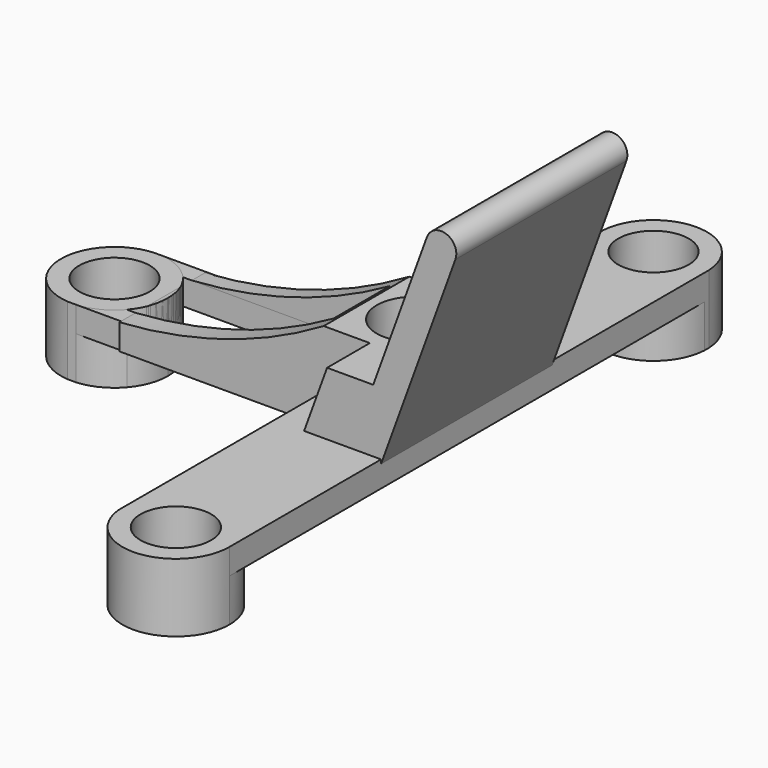
from build123d import *

# Parameters (mm, degrees)
F0_R      = 2.286
F0_R_2    = 2.0955
F2_DEPTH  = 1.524
F3_DEPTH  = 6.35
F4_DEPTH  = 3.175
F5_DEPTH  = 1.524
F6_DEPTH  = 12.7
F0_R_3    = 0.8255
F7_DEPTH  = 2.54
F8_DEPTH  = 1.524
F9_DEPTH  = 2.54
F10_DEPTH = 1.524
F11_DEPTH = 2.54
F12_DEPTH = 1.524
F13_DEPTH = 25.4


with BuildPart() as f2:
    # F0 (on Top) → F2 (new body)
    with BuildSketch(Plane.XY):
        with BuildLine():
            Line((4.9948175588, 3.2833689949), (4.9948175588, 2.2014643259))
            Line((4.9948175588, 2.2014643259), (4.9948175588, -1.9667148894))
            Line((4.9948175588, -1.9667148894), (4.9948175588, -3.0515958757))
            Line((4.9948175588, -3.0515958757), (4.9948175588, -17.3166585326))
            ThreePointArc((4.9948175588, -17.3166585326), (8.3062650536, -14.4464316119), (11.3304992405, -17.6178500122))
            Line((11.3304992405, -17.6178500122), (11.3304992405, 17.6788508391))
            ThreePointArc((11.3304992405, 17.6788508391), (8.2060050581, 14.6658888438), (4.9948175588, 17.5862790105))
            Line((4.9948175588, 17.5862790105), (4.9948175588, 3.2833689949))
        make_face()
        with Locations((8.2809459418, 0)):
            Circle(F0_R, mode=Mode.SUBTRACT)
        with BuildLine():
            Line((4.9948175588, 18.0948209651), (4.9948175588, 17.5862790105))
            ThreePointArc((4.9948175588, 17.5862790105), (8.2060050581, 14.6658888438), (11.3304992405, 17.6788508391))
            Line((11.3304992405, 17.6788508391), (11.3304992405, 18.0022491365))
            ThreePointArc((11.3304992405, 18.0022491365), (8.2060050581, 21.0152111318), (4.9948175588, 18.0948209651))
        make_face()
        with Locations((8.1596194911, 17.8405499878)):
            Circle(F0_R_2, mode=Mode.SUBTRACT)
        with BuildLine():
            ThreePointArc((11.3304992405, -17.6178500122), (8.3062650536, -14.4464316119), (4.9948175588, -17.3166585326))
            Line((4.9948175588, -17.3166585326), (4.9948175588, -17.9190414918))
            ThreePointArc((4.9948175588, -17.9190414918), (8.3062650536, -20.7892684125), (11.3304992405, -17.6178500122))
        make_face()
        with Locations((8.1554992405, -17.6178500122)):
            Circle(F0_R_2, mode=Mode.SUBTRACT)
    extrude(amount=F2_DEPTH)

    # F1 (on Front) → F3 (join, symmetric)
    with BuildSketch(Plane.XZ):
        with BuildLine():
            Line((10.8624471896, 5.2727888553), (8.1229047444, 5.2727888553))
            Line((8.1229047444, 5.2727888553), (6.2037665495, 0))
            Line((6.2037665495, 0), (10.8624471896, 0))
            Line((10.8624471896, 0), (15.7450092285, 13.4147289508))
            ThreePointArc((15.7450092285, 13.4147289508), (15.2060879556, 14.5704493502), (14.0503675562, 14.0315280773))
            Line((14.0503675562, 14.0315280773), (10.8624471896, 5.2727888553))
        make_face()
    extrude(amount=F3_DEPTH, both=True)

    # F1 (on Front) → F4 (join, symmetric)
    with BuildSketch(Plane.XZ):
        with BuildLine():
            Line((8.1229047444, 5.2727888553), (5.3833622992, 5.2727888553))
            ThreePointArc((5.3833622992, 5.2727888553), (-0.4659601575, 2.6817210776), (-6.7578507587, 1.524))
            Line((-6.7578507587, 1.524), (-6.7578507587, 0))
            Line((-6.7578507587, 0), (5.0566992405, 0))
            Line((5.0566992405, 0), (6.2037665495, 0))
            Line((6.2037665495, 0), (8.1229047444, 5.2727888553))
        make_face()
    extrude(amount=F4_DEPTH, both=True)

    # F0 (on Top) → F6 (cut, symmetric)
    with BuildSketch(Plane.XY):
        with BuildLine():
            ThreePointArc((-7.2838490429, 2.2014643259), (-6.7026349357, 1.2283188177), (-6.5003007595, 0.1130238343))
            ThreePointArc((-6.5003007595, 0.1130238343), (-6.7006139401, -0.9968695509), (-7.2762776581, -1.9667148894))
            Line((-7.2762776581, -1.9667148894), (4.9948175588, -1.9667148894))
            Line((4.9948175588, -1.9667148894), (4.9948175588, 2.2014643259))
            Line((4.9948175588, 2.2014643259), (-7.2838490429, 2.2014643259))
        make_face()
    extrude(amount=F6_DEPTH, both=True, mode=Mode.SUBTRACT)

    # F0 (on Top) → F7 (join)
    with BuildSketch(Plane.XY):
        with BuildLine():
            ThreePointArc((11.3304992405, -17.6178500122), (8.3062650536, -14.4464316119), (4.9948175588, -17.3166585326))
            Line((4.9948175588, -17.3166585326), (4.9948175588, -17.9190414918))
            ThreePointArc((4.9948175588, -17.9190414918), (8.3062650536, -20.7892684125), (11.3304992405, -17.6178500122))
        make_face()
        with Locations((8.1554992405, -17.6178500122)):
            Circle(F0_R_2, mode=Mode.SUBTRACT)
        with Locations((8.1554992405, -17.6178500122)):
            Circle(F0_R_2)
        with Locations((8.1554992405, -17.6178500122)):
            Circle(F0_R_3, mode=Mode.SUBTRACT)
    extrude(amount=-F7_DEPTH)

    # F0 (on Top) → F8 (cut)
    with BuildSketch(Plane.XY):
        with Locations((8.1554992405, -17.6178500122)):
            Circle(F0_R_2)
        with Locations((8.1554992405, -17.6178500122)):
            Circle(F0_R_3, mode=Mode.SUBTRACT)
    extrude(amount=-F8_DEPTH, mode=Mode.SUBTRACT)

    # F0 (on Top) → F11 (join)
    with BuildSketch(Plane.XY):
        with BuildLine():
            Line((4.9948175588, 18.0948209651), (4.9948175588, 17.5862790105))
            ThreePointArc((4.9948175588, 17.5862790105), (8.2060050581, 14.6658888438), (11.3304992405, 17.6788508391))
            Line((11.3304992405, 17.6788508391), (11.3304992405, 18.0022491365))
            ThreePointArc((11.3304992405, 18.0022491365), (8.2060050581, 21.0152111318), (4.9948175588, 18.0948209651))
        make_face()
        with Locations((8.1596194911, 17.8405499878)):
            Circle(F0_R_2, mode=Mode.SUBTRACT)
        with Locations((8.1596194911, 17.8405499878)):
            Circle(F0_R_2)
        with Locations((8.1596194911, 17.8405499878)):
            Circle(F0_R_3, mode=Mode.SUBTRACT)
    extrude(amount=-F11_DEPTH)

    # F0 (on Top) → F12 (cut)
    with BuildSketch(Plane.XY):
        with Locations((8.1596194911, 17.8405499878)):
            Circle(F0_R_2)
        with Locations((8.1596194911, 17.8405499878)):
            Circle(F0_R_3, mode=Mode.SUBTRACT)
    extrude(amount=-F12_DEPTH, mode=Mode.SUBTRACT)

    # F0 (on Top) → F13 (cut)
    with BuildSketch(Plane.XY):
        with Locations((8.2809459418, 0)):
            Circle(F0_R)
    extrude(amount=F13_DEPTH, mode=Mode.SUBTRACT)


with BuildPart() as f2b:
    # F0 (on Top) → F2, piece 2 (new body)
    with BuildSketch(Plane.XY):
        with BuildLine():
            ThreePointArc((-7.2762776581, -1.9667148894), (-6.7006139401, -0.9968695509), (-6.5003007595, 0.1130238343))
            ThreePointArc((-6.5003007595, 0.1130238343), (-6.7026349357, 1.2283188177), (-7.2838490429, 2.2014643259))
            ThreePointArc((-7.2838490429, 2.2014643259), (-8.2841595771, 2.9670300029), (-9.5034387136, 3.2833689949))
            Line((-9.5034387136, 3.2833689949), (-9.8471628054, 3.2833689949))
            ThreePointArc((-9.8471628054, 3.2833689949), (-12.8500172326, 0.1554539585), (-9.9318296879, -3.0515958757))
            Line((-9.9318296879, -3.0515958757), (-9.4187718311, -3.0515958757))
            ThreePointArc((-9.4187718311, -3.0515958757), (-8.2409957591, -2.7195358148), (-7.2762776581, -1.9667148894))
        make_face()
        with Locations((-9.6753007595, 0.1130238343)):
            Circle(F0_R_2, mode=Mode.SUBTRACT)
    extrude(amount=F2_DEPTH)

    # F0 (on Top) → F9 (join)
    with BuildSketch(Plane.XY):
        with BuildLine():
            ThreePointArc((-7.2762776581, -1.9667148894), (-6.7006139401, -0.9968695509), (-6.5003007595, 0.1130238343))
            ThreePointArc((-6.5003007595, 0.1130238343), (-6.7026349357, 1.2283188177), (-7.2838490429, 2.2014643259))
            ThreePointArc((-7.2838490429, 2.2014643259), (-8.2841595771, 2.9670300029), (-9.5034387136, 3.2833689949))
            Line((-9.5034387136, 3.2833689949), (-9.8471628054, 3.2833689949))
            ThreePointArc((-9.8471628054, 3.2833689949), (-12.8500172326, 0.1554539585), (-9.9318296879, -3.0515958757))
            Line((-9.9318296879, -3.0515958757), (-9.4187718311, -3.0515958757))
            ThreePointArc((-9.4187718311, -3.0515958757), (-8.2409957591, -2.7195358148), (-7.2762776581, -1.9667148894))
        make_face()
        with Locations((-9.6753007595, 0.1130238343)):
            Circle(F0_R_2, mode=Mode.SUBTRACT)
        with Locations((-9.6753007595, 0.1130238343)):
            Circle(F0_R_2)
        with Locations((-9.6753007595, 0.1130238343)):
            Circle(F0_R_3, mode=Mode.SUBTRACT)
    extrude(amount=-F9_DEPTH)

    # F0 (on Top) → F10 (cut)
    with BuildSketch(Plane.XY):
        with Locations((-9.6753007595, 0.1130238343)):
            Circle(F0_R_2)
        with Locations((-9.6753007595, 0.1130238343)):
            Circle(F0_R_3, mode=Mode.SUBTRACT)
    extrude(amount=-F10_DEPTH, mode=Mode.SUBTRACT)


with BuildPart() as f5:
    # F0 (on Top) → F5 (new body)
    with BuildSketch(Plane.XY):
        with BuildLine():
            ThreePointArc((-9.5034387136, 3.2833689949), (-8.2841595771, 2.9670300029), (-7.2838490429, 2.2014643259))
            Line((-7.2838490429, 2.2014643259), (4.9948175588, 2.2014643259))
            Line((4.9948175588, 2.2014643259), (4.9948175588, 3.2833689949))
            Line((4.9948175588, 3.2833689949), (-9.5034387136, 3.2833689949))
        make_face()
    extrude(amount=F5_DEPTH)


with BuildPart() as f5b:
    # F0 (on Top) → F5, piece 2 (new body)
    with BuildSketch(Plane.XY):
        with BuildLine():
            Line((4.9948175588, -1.9667148894), (-7.2762776581, -1.9667148894))
            ThreePointArc((-7.2762776581, -1.9667148894), (-8.2409957591, -2.7195358148), (-9.4187718311, -3.0515958757))
            Line((-9.4187718311, -3.0515958757), (4.9948175588, -3.0515958757))
            Line((4.9948175588, -3.0515958757), (4.9948175588, -1.9667148894))
        make_face()
    extrude(amount=F5_DEPTH)


solid = Compound([f2.part, f2b.part, f5.part, f5b.part])
